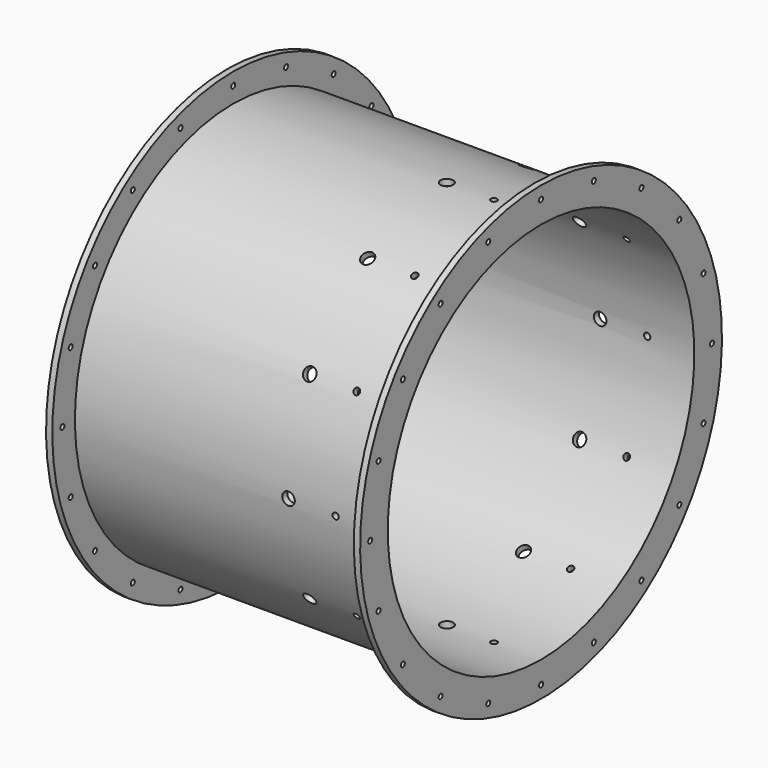
from build123d import *

# Parameters (mm, degrees)
F2_R            = 4
F3_DEPTH        = 500.001
F3_COPIES_COUNT = 20
F4_R            = 10
F4_R_2          = 5
F5_DEPTH        = 360.001
F5_COPIES_COUNT = 12


# Not quite as in the source:
# - a pattern or mirror of a feature is missing from the dataset's text; its kind, count and spacing are read off the source's solid


with BuildPart() as f1:
    # F0 (on Front) → F1 (revolve)
    with BuildSketch(Plane.XZ):
        Polygon((-250, 305), (0, 305), (250, 305), (250, 360), (240, 360), (240, 315), (0, 315), (-240, 315), (-240, 360), (-250, 360), align=None)
    revolve(axis=Axis((125, 0, 0), (1, 0, 0)))

    # F2 (on face) → F3 (cut, through all)
    with BuildSketch(Plane.YZ.offset(250)):
        with Locations((0, 340)):
            Circle(F2_R)
    f3 = extrude(amount=-F3_DEPTH, mode=Mode.SUBTRACT)

    # F3_copies: F3 ×20 about axis
    f3_copies_axis = Axis((0, 0, 0), (1, 0, 0))
    for i in range(1, F3_COPIES_COUNT):
        add(f3.rotate(f3_copies_axis, i * 360 / F3_COPIES_COUNT), mode=Mode.SUBTRACT)

    # F4 (on Top) → F5 (cut, through all)
    with BuildSketch(Plane.XY):
        with Locations((100, 0)):
            Circle(F4_R)
        with Locations((175, 0)):
            Circle(F4_R_2)
    f5 = extrude(amount=-F5_DEPTH, mode=Mode.SUBTRACT)

    # F5_copies: F5 ×12 about axis
    f5_copies_axis = Axis((0, 0, 0), (1, 0, 0))
    for i in range(1, F5_COPIES_COUNT):
        add(f5.rotate(f5_copies_axis, i * 360 / F5_COPIES_COUNT), mode=Mode.SUBTRACT)


solid = f1.part
